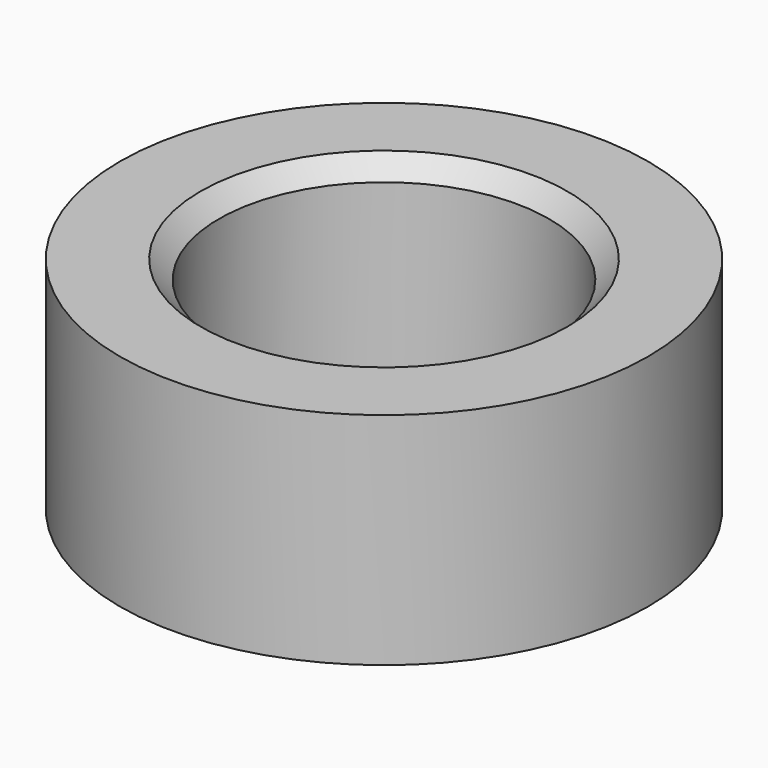
from build123d import *

# Parameters (mm, degrees)
F0_R     = 7.2
F0_R_2   = 4.5
F2_DEPTH = 6
F3_SIZE2 = 0.5
F3_SIZE  = 0.5
F4_SIZE2 = 0.5
F4_SIZE  = 0.5


# Not quite as in the source:
# - the program builds the solid bodies; features that only make, move or delete a surface that nothing else refers to are left out


with BuildPart() as f2:
    # F0 (on Top) → F2 (new body)
    with BuildSketch(Plane.XY):
        Circle(F0_R)
        Circle(F0_R_2, mode=Mode.SUBTRACT)
    extrude(amount=F2_DEPTH)

    # F3
    f3_edges = [f2.edges().sort_by_distance(p)[0] for p in [
        (-4.5, 0, 0),
    ]]
    chamfer(f3_edges, length=F3_SIZE, length2=F3_SIZE2)

    # F4
    f4_edges = [f2.edges().sort_by_distance(p)[0] for p in [
        (-4.5, 0, 6),
    ]]
    chamfer(f4_edges, length=F4_SIZE, length2=F4_SIZE2)


solid = f2.part
